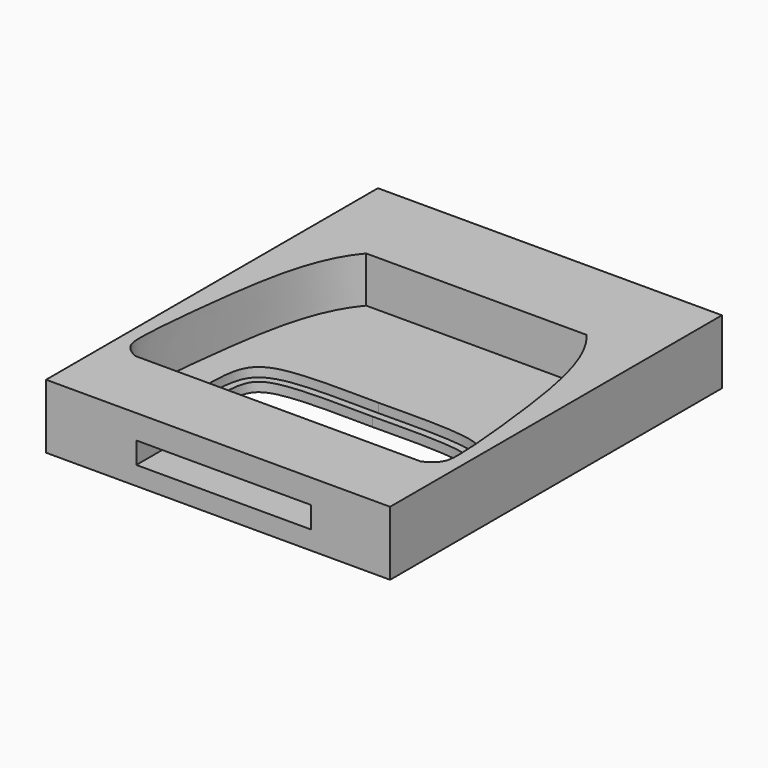
from build123d import *

# Parameters (mm, degrees)
F0_W       = 37.4453663826
F0_H       = 45.1489761472
F1_DEPTH   = 7
F2_W       = 19
F2_H       = 2.3503608536
F3_DEPTH   = 5
F1_FACE2_W = 37.4453663826
F1_FACE2_H = 45.1489761472
F5_DEPTH   = 5
F7_DEPTH   = 1
F8_DEPTH   = 25


# Not quite as in the source:
# - the dataset's text gives a spline's control points without its knots; the knots are read off the source's solid


with BuildPart() as f1:
    # F0 (on Top) → F1 (new body)
    with BuildSketch(Plane.XY):
        Rectangle(F0_W, F0_H)
    extrude(amount=F1_DEPTH)

    # F2 (on face) → F3 (cut)
    with BuildSketch(Plane.XZ.offset(22.5744880736)):
        with Locations((0.6016407423, 3.201102023)):
            Rectangle(F2_W, F2_H)
    extrude(amount=-F3_DEPTH, mode=Mode.SUBTRACT)

    # F4 (on face) + F1_face2 (on face) → F5 (cut)
    with BuildSketch(Plane.XY.offset(7)):
        with BuildLine():
            add(Edge.make_bspline(
                [(12, 12.5702119679), (13.3253792301, 11.0086901113), (15.2358497186, 6.7812120759), (16.5545280862, -1.951122829), (17.4806651469, -11.2851763765), (17.1494033542, -13.4820758702), (15.8976428149, -14.3024219384), (15.5, -14.4297880321)],
                knots=[0, 0, 0, 0, 0.2223639885, 0.4930350124, 0.7613325305, 0.8867013323, 1, 1, 1, 1], degree=3))
            Line((12, 12.5702119679), (0, 12.5702119679))
            Line((0, 12.5702119679), (-12, 12.5702119679))
            add(Edge.make_bspline(
                [(-12, 12.5702119679), (-13.3253792301, 11.0086901113), (-15.2358497186, 6.7812120759), (-16.5545280862, -1.951122829), (-17.4806651469, -11.2851763765), (-17.1494033542, -13.4820758702), (-15.8976428149, -14.3024219384), (-15.5, -14.4297880321)],
                knots=[0, 0, 0, 0, 0.2223639885, 0.4930350124, 0.7613325305, 0.8867013323, 1, 1, 1, 1], degree=3))
            Line((-15.5, -14.4297880321), (0, -14.4297880321))
            Line((0, -14.4297880321), (15.5, -14.4297880321))
        make_face()
    with BuildSketch(Plane(origin=(0, 0, 0), x_dir=(1, 0, 0), z_dir=(0, 0, -1))):
        Rectangle(F1_FACE2_W, F1_FACE2_H)
    extrude(amount=-F5_DEPTH, dir=(0, 0, 1), mode=Mode.SUBTRACT)

    # F6 (on face) → F7 (cut)
    with BuildSketch(Plane.XY.offset(2)):
        with BuildLine():
            add(Edge.make_bspline(
                [(0, -13.7379904656), (-6.143513217, -13.6393481481), (-14.1599602379, -13.7321618792), (-13.265150625, -9.1725055801), (-13.8515294472, -2.1039104698), (-8.7024669299, -0.5093012378), (-2.7921305831, -0.741491258), (0, -0.7379904656)],
                knots=[0, 0, 0, 0, 0.2784276458, 0.4147120098, 0.6092064296, 0.7707712857, 1, 1, 1, 1], degree=3))
            add(Edge.make_bspline(
                [(0, -13.7379904656), (6.143513217, -13.6393481481), (14.1599602379, -13.7321618792), (13.265150625, -9.1725055801), (13.8515294472, -2.1039104698), (8.7024669299, -0.5093012378), (2.7921305831, -0.741491258), (0, -0.7379904656)],
                knots=[0, 0, 0, 0, 0.2784276458, 0.4147120098, 0.6092064296, 0.7707712857, 1, 1, 1, 1], degree=3))
        make_face()
        with BuildLine():
            add(Edge.make_bspline(
                [(0, -12.9378874867), (1.3774219447, -12.9158171677), (3.3833255401, -12.8947560137), (5.8256959578, -12.8370443978), (7.5145271403, -12.7656213856), (9.0276107381, -12.6533856445), (10.3321294547, -12.4890755572), (11.2135820807, -12.3021291271), (11.7709631592, -12.1252953157), (12.1073406956, -11.983466617), (12.3564668909, -11.8391696547), (12.5105234515, -11.7108897101), (12.600900341, -11.5971923014), (12.6679648826, -11.4673867456), (12.720664906, -11.2910950306), (12.7664963954, -10.9732099903), (12.7660010847, -10.4193684462), (12.7171849981, -9.6943166542), (12.6914362795, -9.0206172469), (12.6814730621, -8.3233976346), (12.6825982166, -7.4161857043), (12.6725900892, -6.3166706104), (12.6186607671, -5.2583936291), (12.4928373078, -4.3005164272), (12.3110364451, -3.6399402975), (12.1253666084, -3.2312247276), (11.9125327284, -2.8948065244), (11.5808934895, -2.5562440652), (11.0390168629, -2.2301617142), (10.3272024925, -1.9755236276), (9.4575986645, -1.7918299667), (8.4481657144, -1.6645005524), (6.9664260364, -1.5509991752), (4.931288851, -1.5008643816), (2.3956919954, -1.5199786925), (0.7683085646, -1.5389453427), (0, -1.5379911665)],
                knots=[0.0001936351, 0.0001936351, 0.0001936351, 0.0001936351, 0.0625, 0.09375, 0.125, 0.15625, 0.1875, 0.21875, 0.234375, 0.25, 0.265625, 0.28125, 0.296875, 0.3125, 0.328125, 0.34375, 0.375, 0.40625, 0.421875, 0.4375, 0.46875, 0.5, 0.53125, 0.5625, 0.59375, 0.609375, 0.625, 0.65625, 0.6875, 0.71875, 0.75, 0.78125, 0.8125, 0.875, 0.9375, 0.9999728127, 0.9999728127, 0.9999728127, 0.9999728127], degree=3))
            add(Edge.make_bspline(
                [(0, -12.9378874867), (-1.3774219447, -12.9158171677), (-3.3833255401, -12.8947560137), (-5.8256959578, -12.8370443978), (-7.5145271403, -12.7656213856), (-9.0276107381, -12.6533856445), (-10.3321294547, -12.4890755572), (-11.2135820807, -12.3021291271), (-11.7709631592, -12.1252953157), (-12.1073406956, -11.983466617), (-12.3564668909, -11.8391696547), (-12.5105234515, -11.7108897101), (-12.600900341, -11.5971923014), (-12.6679648826, -11.4673867456), (-12.720664906, -11.2910950306), (-12.7664963954, -10.9732099903), (-12.7660010847, -10.4193684462), (-12.7171849981, -9.6943166542), (-12.6914362795, -9.0206172469), (-12.6814730621, -8.3233976346), (-12.6825982166, -7.4161857043), (-12.6725900892, -6.3166706104), (-12.6186607671, -5.2583936291), (-12.4928373078, -4.3005164272), (-12.3110364451, -3.6399402975), (-12.1253666084, -3.2312247276), (-11.9125327284, -2.8948065244), (-11.5808934895, -2.5562440652), (-11.0390168629, -2.2301617142), (-10.3272024925, -1.9755236276), (-9.4575986645, -1.7918299667), (-8.4481657144, -1.6645005524), (-6.9664260364, -1.5509991752), (-4.931288851, -1.5008643816), (-2.3956919954, -1.5199786925), (-0.7683085646, -1.5389453427), (0, -1.5379911665)],
                knots=[0.0001936351, 0.0001936351, 0.0001936351, 0.0001936351, 0.0625, 0.09375, 0.125, 0.15625, 0.1875, 0.21875, 0.234375, 0.25, 0.265625, 0.28125, 0.296875, 0.3125, 0.328125, 0.34375, 0.375, 0.40625, 0.421875, 0.4375, 0.46875, 0.5, 0.53125, 0.5625, 0.59375, 0.609375, 0.625, 0.65625, 0.6875, 0.71875, 0.75, 0.78125, 0.8125, 0.875, 0.9375, 0.9999728127, 0.9999728127, 0.9999728127, 0.9999728127], degree=3))
        make_face(mode=Mode.SUBTRACT)
    extrude(amount=-F7_DEPTH, mode=Mode.SUBTRACT)

    # F8 (cut): a face of the model
    f8_faces = [f1.faces().sort_by_distance(p)[0] for p in [
        (0, -7.2433932356, 2),
    ]]
    extrude(f8_faces, amount=-F8_DEPTH, mode=Mode.SUBTRACT)


solid = f1.part
